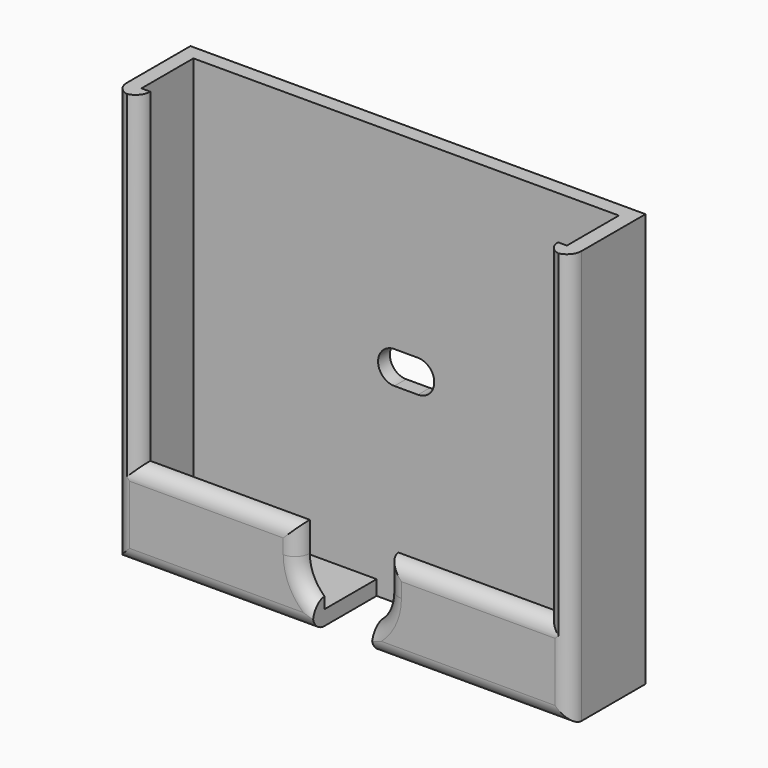
from build123d import *

# Parameters (mm, degrees)
F0_W         = 77
F0_H         = 70
F1_DEPTH     = 8
F2_T         = -2.5
F4_DEPTH     = 13.5
F6_DEPTH     = 2.5
F7_T1_DEPTH  = 82.5
F7_T3_DEPTH  = 46
F7_T5_DEPTH  = 46
F7_T7_DEPTH  = 33.25
F7_T9_DEPTH  = 33.25
F7_T11_DEPTH = 61.25
F7_T13_DEPTH = 11.25
F7_T16_ANGLE = 95.9416658211
F7_T18_ANGLE = 95.9416658211
F7_T23_DEPTH = 39.5
F7_T27_DEPTH = 67.5
F7_T34_DEPTH = 67.5
F7_T38_DEPTH = 39.5


# Not quite as in the source:
# - a fillet or chamfer that OpenCascade refuses, or shapes differently, is made with other operations: its cross-section is extruded or revolved along the edge and cut away or added


with BuildPart() as f1:
    # F0 (on Front) → F1 (new body, symmetric)
    with BuildSketch(Plane.XZ):
        Rectangle(F0_W, F0_H)
    extrude(amount=F1_DEPTH, both=True)

    # F2
    f2_openings = [f1.faces().sort_by_distance(p)[0] for p in [
        (0, 0, 35),
    ]]
    offset(amount=F2_T, openings=f2_openings)

    # F3 (on face) → F4 (cut, through all)
    with BuildSketch(Plane.XZ.offset(8)):
        Polygon((34.5, 35), (-34.5, 35), (-34.5, -20), (-7.5, -20), (7.5, -20), (34.5, -20), align=None)
        with BuildLine():
            Line((7.5, -20), (-7.5, -20))
            Line((-7.5, -20), (-7.5, -25))
            ThreePointArc((-7.5, -25), (-6.8465319688, -28.0618621785), (-5, -30.5901699437))
            ThreePointArc((-5, -30.5901699437), (0, -32.5), (5, -30.5901699437))
            ThreePointArc((5, -30.5901699437), (6.8465319688, -28.0618621785), (7.5, -25))
            Line((7.5, -25), (7.5, -20))
        make_face()
        with BuildLine():
            Line((-5, -30.5901699437), (-5, -35))
            Line((-5, -35), (5, -35))
            Line((5, -35), (5, -30.5901699437))
            ThreePointArc((5, -30.5901699437), (0, -32.5), (-5, -30.5901699437))
        make_face()
    extrude(amount=-F4_DEPTH, mode=Mode.SUBTRACT)

    # F5 (on face) → F6 (cut, through all)
    with BuildSketch(Plane(origin=(0, 8, 0), x_dir=(-1, 0, 0), z_dir=(0, 1, 0))):
        with BuildLine():
            ThreePointArc((2, -2.75), (4.75, 0), (2, 2.75))
            Line((2, 2.75), (-2, 2.75))
            ThreePointArc((-2, 2.75), (-4.75, 0), (-2, -2.75))
            Line((-2, -2.75), (2, -2.75))
        make_face()
    extrude(amount=-F6_DEPTH, mode=Mode.SUBTRACT)

    # F7: fillet of radius 2.5 on 10 edges, made by hand

    # F7_s2 → F7_t1 (cut)
    with BuildSketch(Plane.XY.offset(-41.25)):
        with BuildLine():
            ThreePointArc((38.5, -5.5), (37.767766953, -7.267766953), (36, -8))
            Line((36, -8), (38.5, -8))
            Line((38.5, -8), (38.5, -5.5))
        make_face()
        with BuildLine():
            ThreePointArc((-38.5, -5.5), (-37.767766953, -7.267766953), (-36, -8))
            Line((-36, -8), (-38.5, -8))
            Line((-38.5, -8), (-38.5, -5.5))
        make_face()
    extrude(amount=F7_T1_DEPTH, mode=Mode.SUBTRACT)

    # F7_s4 → F7_t3 (cut)
    with BuildSketch(Plane.YZ.offset(-44.75)):
        with BuildLine():
            ThreePointArc((-5.5, -35), (-7.267766953, -34.267766953), (-8, -32.5))
            Line((-8, -32.5), (-8, -35))
            Line((-8, -35), (-5.5, -35))
        make_face()
    extrude(amount=F7_T3_DEPTH, mode=Mode.SUBTRACT)

    # F7_s6 → F7_t5 (cut)
    with BuildSketch(Plane.YZ.offset(-1.25)):
        with BuildLine():
            ThreePointArc((-8, -32.5), (-7.267766953, -34.267766953), (-5.5, -35))
            Line((-5.5, -35), (-8, -35))
            Line((-8, -35), (-8, -32.5))
        make_face()
    extrude(amount=F7_T5_DEPTH, mode=Mode.SUBTRACT)

    # F7_s8 → F7_t7 (cut)
    with BuildSketch(Plane.YZ.offset(1.25)):
        with BuildLine():
            ThreePointArc((-8, -22.5), (-7.267766953, -20.732233047), (-5.5, -20))
            Line((-5.5, -20), (-8, -20))
            Line((-8, -20), (-8, -22.5))
        make_face()
    extrude(amount=F7_T7_DEPTH, mode=Mode.SUBTRACT)

    # F7_s10 → F7_t9 (cut)
    with BuildSketch(Plane.YZ.offset(-34.5)):
        with BuildLine():
            ThreePointArc((-8, -22.5), (-7.267766953, -20.732233047), (-5.5, -20))
            Line((-5.5, -20), (-8, -20))
            Line((-8, -20), (-8, -22.5))
        make_face()
    extrude(amount=F7_T9_DEPTH, mode=Mode.SUBTRACT)

    # F7_s12 → F7_t11 (cut)
    with BuildSketch(Plane.XY.offset(-20)):
        with BuildLine():
            ThreePointArc((37, -8), (35.232233047, -7.267766953), (34.5, -5.5))
            Line((34.5, -5.5), (34.5, -8))
            Line((34.5, -8), (37, -8))
        make_face()
        with BuildLine():
            ThreePointArc((-37, -8), (-35.232233047, -7.267766953), (-34.5, -5.5))
            Line((-34.5, -5.5), (-34.5, -8))
            Line((-34.5, -8), (-37, -8))
        make_face()
    extrude(amount=F7_T11_DEPTH, mode=Mode.SUBTRACT)

    # F7_s14 → F7_t13 (cut)
    with BuildSketch(Plane.XY.offset(-25)):
        with BuildLine():
            ThreePointArc((10, -8), (8.232233047, -7.267766953), (7.5, -5.5))
            Line((7.5, -5.5), (7.5, -8))
            Line((7.5, -8), (10, -8))
        make_face()
        with BuildLine():
            ThreePointArc((-10, -8), (-8.232233047, -7.267766953), (-7.5, -5.5))
            Line((-7.5, -5.5), (-7.5, -8))
            Line((-7.5, -8), (-10, -8))
        make_face()
    extrude(amount=F7_T13_DEPTH, mode=Mode.SUBTRACT)

    # F7_s15 → F7_t16 (revolve, cut)
    with BuildSketch(Plane.XY.offset(-25)):
        with BuildLine():
            ThreePointArc((-10, -8), (-8.232233047, -7.267766953), (-7.5, -5.5))
            Line((-7.5, -5.5), (-7.5, -8))
            Line((-7.5, -8), (-10, -8))
        make_face()
    revolve(axis=Axis((0, -8, -25), (0, -1, 0)), revolution_arc=F7_T16_ANGLE, mode=Mode.SUBTRACT)

    # F7_s17 → F7_t18 (revolve, cut)
    with BuildSketch(Plane(origin=(2.5739938884, 0, -0.2678883482), x_dir=(0, 1, 0), z_dir=(-0.9946278028, 0, 0.1035158632))):
        with BuildLine():
            ThreePointArc((-8, 34.8656950696), (-7.267766953, 33.0979281167), (-5.5, 32.3656950696))
            Line((-5.5, 32.3656950696), (-8, 32.3656950696))
            Line((-8, 32.3656950696), (-8, 34.8656950696))
        make_face()
    revolve(axis=Axis((0, -8, -25), (0, -1, 0)), revolution_arc=F7_T18_ANGLE, mode=Mode.SUBTRACT)


with BuildPart() as f7_tool21:
    # F7_s22 → F7_t23 (new body)
    with BuildSketch(Plane.YZ.offset(1.25)):
        with BuildLine():
            ThreePointArc((-8, -22.5), (-7.267766953, -20.732233047), (-5.5, -20))
            Line((-5.5, -20), (-8, -20))
            Line((-8, -20), (-8, -22.5))
        make_face()
    extrude(amount=F7_T23_DEPTH)

    split(bisect_by=Plane.YZ.offset(34.5), keep=Keep.TOP)


with BuildPart() as f7_tool25:
    # F7_s26 → F7_t27 (new body)
    with BuildSketch(Plane.XY.offset(-26.25)):
        with BuildLine():
            ThreePointArc((37, -8), (35.232233047, -7.267766953), (34.5, -5.5))
            Line((34.5, -5.5), (34.5, -8))
            Line((34.5, -8), (37, -8))
        make_face()
    extrude(amount=F7_T27_DEPTH)

    split(bisect_by=Plane.XY.offset(-20), keep=Keep.BOTTOM)


with BuildPart() as f7_tool21_1:
    add(f7_tool21.part)

    # F7_t29: intersect F7_tool25
    add(f7_tool25.part, mode=Mode.INTERSECT)


with BuildPart() as f1_1:
    add(f1.part)

    # F7_t19: cut F7_tool21
    add(f7_tool21_1.part, mode=Mode.SUBTRACT)


with BuildPart() as f7_tool32:
    # F7_s33 → F7_t34 (new body)
    with BuildSketch(Plane.XY.offset(41.25)):
        with BuildLine():
            ThreePointArc((-37, -8), (-35.232233047, -7.267766953), (-34.5, -5.5))
            Line((-34.5, -5.5), (-34.5, -8))
            Line((-34.5, -8), (-37, -8))
        make_face()
    extrude(amount=-F7_T34_DEPTH)

    split(bisect_by=Plane.XY.offset(-20), keep=Keep.BOTTOM)


with BuildPart() as f7_tool36:
    # F7_s37 → F7_t38 (new body)
    with BuildSketch(Plane.YZ.offset(-40.75)):
        with BuildLine():
            ThreePointArc((-8, -22.5), (-7.267766953, -20.732233047), (-5.5, -20))
            Line((-5.5, -20), (-8, -20))
            Line((-8, -20), (-8, -22.5))
        make_face()
    extrude(amount=F7_T38_DEPTH)

    split(bisect_by=Plane.YZ.offset(-34.5), keep=Keep.BOTTOM)


with BuildPart() as f7_tool32_1:
    add(f7_tool32.part)

    # F7_t40: intersect F7_tool36
    add(f7_tool36.part, mode=Mode.INTERSECT)


with BuildPart() as f1_2:
    add(f1_1.part)

    # F7_t30: cut F7_tool32
    add(f7_tool32_1.part, mode=Mode.SUBTRACT)


solid = f1_2.part
